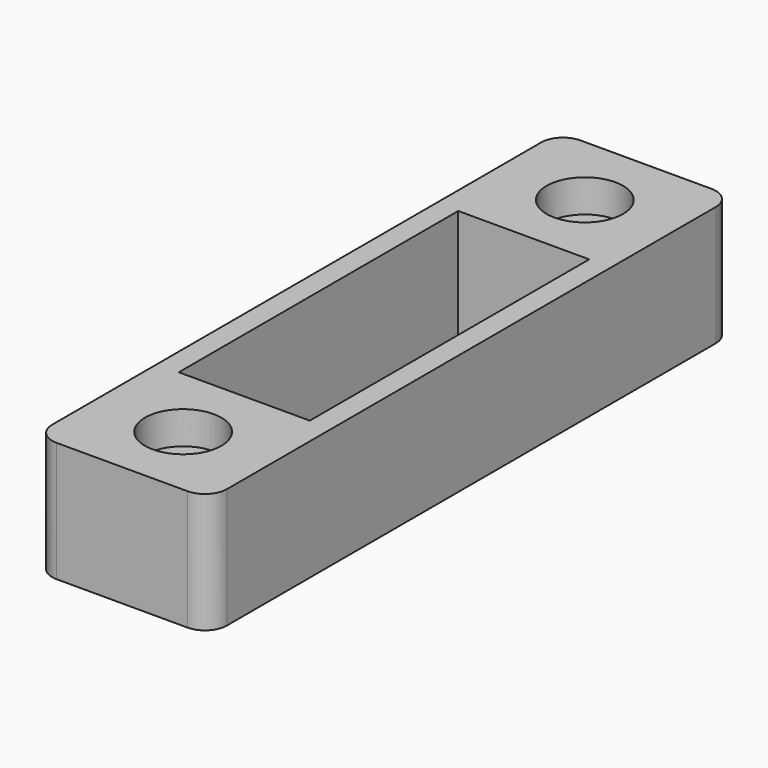
from build123d import *

# Parameters (mm, degrees)
F1_DEPTH = 17.4625
F3_R     = 1.984375
F4_DEPTH = 17.4635
F5_DEPTH = 3.175
F6_R     = 1.984375
F7_DEPTH = 11.1125
F8_R     = 5.55625
F8_R_2   = 1.984375
F9_DEPTH = 4.7625


with BuildPart() as f1:
    # F0 (on Top) → F1 (new body)
    with BuildSketch(Plane.XY):
        with BuildLine():
            Line((22.225, 0), (3.175, 0))
            ThreePointArc((3.175, 0), (0.9299359697, -0.9299359697), (0, -3.175))
            Line((0, -3.175), (0, -92.075))
            ThreePointArc((0, -92.075), (0.9299359697, -94.3200640303), (3.175, -95.25))
            Line((3.175, -95.25), (22.225, -95.25))
            ThreePointArc((22.225, -95.25), (24.4700640303, -94.3200640303), (25.4, -92.075))
            Line((25.4, -92.075), (25.4, -3.175))
            ThreePointArc((25.4, -3.175), (24.4700640303, -0.9299359697), (22.225, 0))
        make_face()
        Polygon((3.175, -22.225), (12.7, -22.225), (22.225, -22.225), (22.225, -47.625), (22.225, -73.025), (12.7, -73.025), (3.175, -73.025), (3.175, -47.625), align=None, mode=Mode.SUBTRACT)
    extrude(amount=F1_DEPTH)

    # F3 (on face) → F4 (cut, through all)
    with BuildSketch(Plane(origin=(0, 0, 0), x_dir=(1, 0, 0), z_dir=(0, 0, -1))):
        with Locations((12.7, 11.1125)):
            Circle(F3_R)
        with Locations((12.7, 84.1375)):
            Circle(F3_R)
    extrude(amount=-F4_DEPTH, mode=Mode.SUBTRACT)

    # F0 (on Top) → F5 (cut)
    with BuildSketch(Plane.XY):
        Polygon((22.225, -22.225), (12.7, -22.225), (3.175, -22.225), (3.175, -47.625), (3.175, -73.025), (12.7, -73.025), (22.225, -73.025), (22.225, -47.625), align=None)
    extrude(amount=F5_DEPTH, mode=Mode.SUBTRACT)

    # F6 (on face) → F7 (cut)
    with BuildSketch(Plane(origin=(0, 0, 0), x_dir=(1, 0, 0), z_dir=(0, 0, -1))):
        with BuildLine():
            ThreePointArc((11.90625, 80.6549360088), (9.128125, 84.1375), (11.90625, 87.6200639912))
            Line((11.90625, 87.6200639912), (11.90625, 93.6625))
            Line((11.90625, 93.6625), (3.175, 93.6625))
            ThreePointArc((3.175, 93.6625), (2.0524679849, 93.1975320151), (1.5875, 92.075))
            Line((1.5875, 92.075), (1.5875, 74.6125))
            Line((1.5875, 74.6125), (11.90625, 74.6125))
            Line((11.90625, 74.6125), (11.90625, 80.6549360088))
        make_face()
        with BuildLine():
            Line((22.225, 93.6625), (13.49375, 93.6625))
            Line((13.49375, 93.6625), (13.49375, 87.6200639912))
            ThreePointArc((13.49375, 87.6200639912), (16.271875, 84.1375), (13.49375, 80.6549360088))
            Line((13.49375, 80.6549360088), (13.49375, 74.6125))
            Line((13.49375, 74.6125), (23.8125, 74.6125))
            Line((23.8125, 74.6125), (23.8125, 92.075))
            ThreePointArc((23.8125, 92.075), (23.3475320151, 93.1975320151), (22.225, 93.6625))
        make_face()
        with BuildLine():
            Line((11.90625, 20.6375), (1.5875, 20.6375))
            Line((1.5875, 20.6375), (1.5875, 3.175))
            ThreePointArc((1.5875, 3.175), (2.0524679849, 2.0524679849), (3.175, 1.5875))
            Line((3.175, 1.5875), (11.90625, 1.5875))
            Line((11.90625, 1.5875), (11.90625, 7.6299360088))
            ThreePointArc((11.90625, 7.6299360088), (9.128125, 11.1125), (11.90625, 14.5950639912))
            Line((11.90625, 14.5950639912), (11.90625, 20.6375))
        make_face()
        with BuildLine():
            Line((23.8125, 3.175), (23.8125, 20.6375))
            Line((23.8125, 20.6375), (13.49375, 20.6375))
            Line((13.49375, 20.6375), (13.49375, 14.5950639912))
            ThreePointArc((13.49375, 14.5950639912), (16.271875, 11.1125), (13.49375, 7.6299360088))
            Line((13.49375, 7.6299360088), (13.49375, 1.5875))
            Line((13.49375, 1.5875), (22.225, 1.5875))
            ThreePointArc((22.225, 1.5875), (23.3475320151, 2.0524679849), (23.8125, 3.175))
        make_face()
        with Locations((12.7, 11.1125)):
            Circle(F6_R)
    extrude(amount=-F7_DEPTH, mode=Mode.SUBTRACT)

    # F8 (on face) → F9 (cut)
    with BuildSketch(Plane.XY.offset(17.4625)):
        with Locations((12.7, -84.1375)):
            Circle(F8_R)
        with Locations((12.7, -84.1375)):
            Circle(F8_R_2, mode=Mode.SUBTRACT)
        with Locations((12.7, -11.1125)):
            Circle(F8_R)
        with Locations((12.7, -11.1125)):
            Circle(F8_R_2, mode=Mode.SUBTRACT)
        with Locations((12.7, -11.1125)):
            Circle(F8_R_2)
    extrude(amount=-F9_DEPTH, mode=Mode.SUBTRACT)


solid = f1.part
